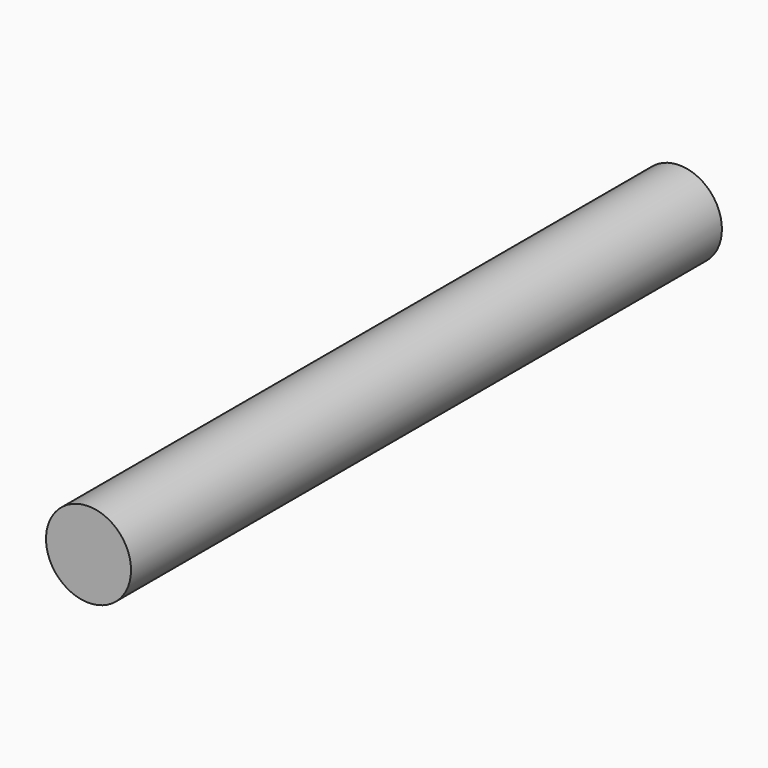
from build123d import *

# Parameters (mm, degrees)
F0_R     = 2.9239691531
F2_DEPTH = 25.4
F3_DEPTH = 25.4


# Not quite as in the source:
# - the program builds the solid bodies; features that only make, move or delete a surface that nothing else refers to are left out


with BuildPart() as f2:
    # F0 (on Front) → F2 (new body)
    with BuildSketch(Plane.XZ):
        with Locations((-12.3839471489, -8.2559641451)):
            Circle(F0_R)
    extrude(amount=F2_DEPTH)

    # F3 (add): a face of the model
    f3_faces = [f2.faces().sort_by_distance(p)[0] for p in [
        (-12.3839471489, -25.4, -8.2559641451),
    ]]
    extrude(f3_faces, amount=F3_DEPTH)


solid = f2.part
